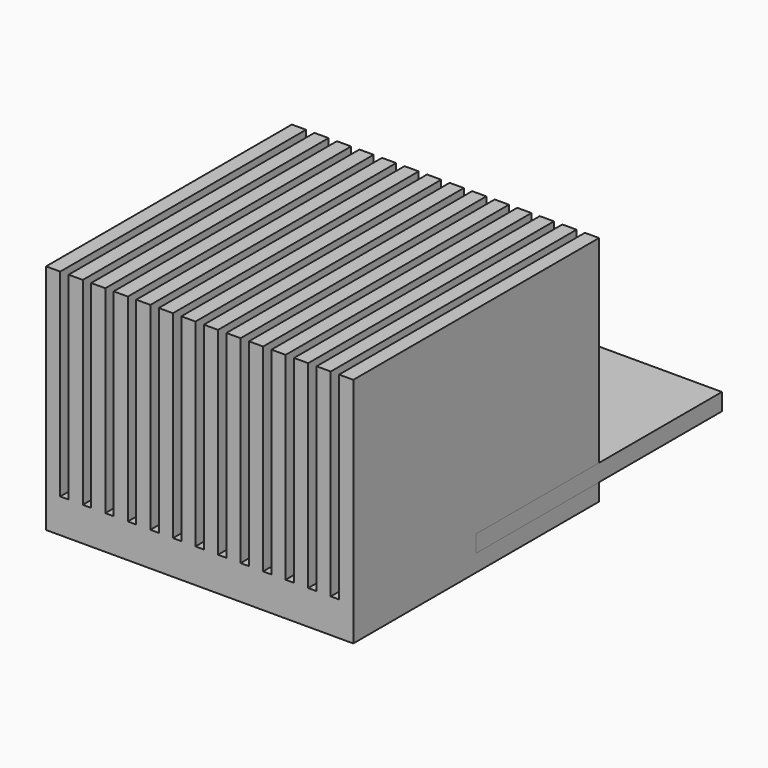
from build123d import *

# Parameters (mm, degrees)
F1_DEPTH = 90
F2_R     = 2
F3_DEPTH = 10.414
F4_W     = 90
F4_H     = 90
F5_DEPTH = 5
F6_R     = 2
F7_DEPTH = 25.4


with BuildPart() as f1:
    # F0 (on Front) → F1 (new body)
    with BuildSketch(Plane.XZ):
        Polygon((-45, 5), (-45, -5), (45, -5), (45, 5), (45, 63), (40.852, 63), (40.852, 5), (38.396, 5), (38.396, 63), (34.248, 63), (34.248, 5), (31.792, 5), (31.792, 63), (27.644, 63), (27.644, 5), (25.188, 5), (25.188, 63), (21.04, 63), (21.04, 5), (18.584, 5), (18.584, 63), (14.436, 63), (14.436, 5), (11.98, 5), (11.98, 63), (7.832, 63), (7.832, 5), (5.376, 5), (5.376, 63), (1.228, 63), (1.228, 5), (-1.228, 5), (-1.228, 63), (-5.376, 63), (-5.376, 5), (-7.832, 5), (-7.832, 63), (-11.98, 63), (-11.98, 5), (-14.436, 5), (-14.436, 63), (-18.584, 63), (-18.584, 5), (-21.04, 5), (-21.04, 63), (-25.188, 63), (-25.188, 5), (-27.644, 5), (-27.644, 63), (-31.792, 63), (-31.792, 5), (-34.248, 5), (-34.248, 63), (-38.396, 63), (-38.396, 5), (-40.852, 5), (-40.852, 63), (-45, 63), align=None)
    extrude(amount=F1_DEPTH)

    # F2 (on face) → F3 (cut)
    with BuildSketch(Plane(origin=(0, 0, -5), x_dir=(1, 0, 0), z_dir=(0, 0, -1))):
        with Locations((0, 45)):
            Circle(F2_R)
    extrude(amount=-F3_DEPTH, mode=Mode.SUBTRACT)


with BuildPart() as f5:
    # F4 (on Top) → F5 (new body)
    with BuildSketch(Plane.XY):
        Rectangle(F4_W, F4_H)
    extrude(amount=F5_DEPTH)

    # F6 (on face) → F7 (cut)
    with BuildSketch(Plane.XY.offset(5)):
        Circle(F6_R)
    extrude(amount=-F7_DEPTH, mode=Mode.SUBTRACT)


solid = Compound([f1.part, f5.part])
